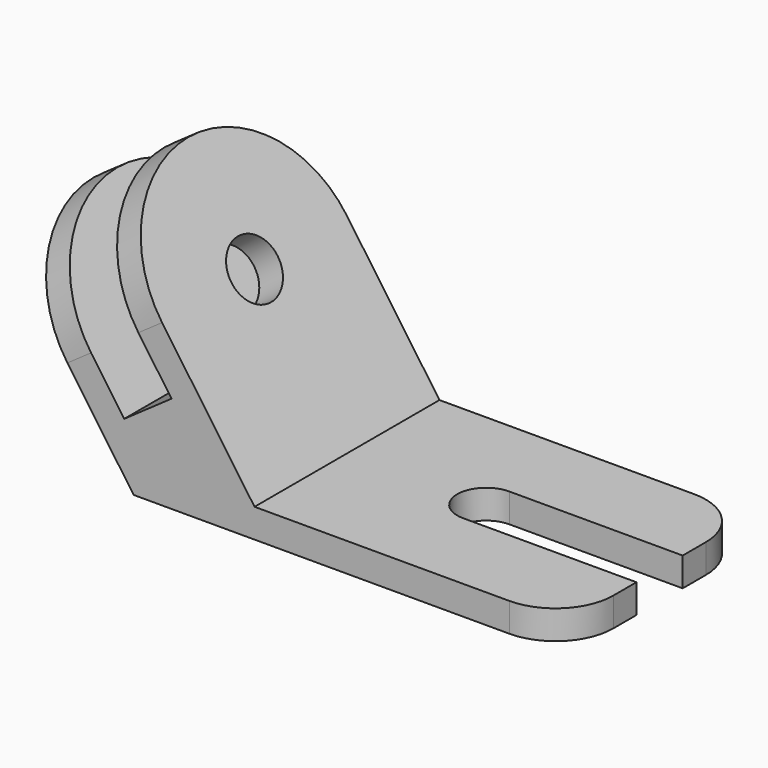
from build123d import *

# Parameters (mm, degrees)
F1_DEPTH = 80
F2_R     = 39.99999
F4_DEPTH = 25
F5_R     = 20
F6_R     = 10
F7_DEPTH = 57.1


# Not quite as in the source:
# - a fillet or chamfer is up to 0.001 mm smaller than in the source, because OpenCascade refuses the exact size


with BuildPart() as f1:
    # F0 (on Front) → F1 (new body)
    with BuildSketch(Plane.XZ):
        Polygon((-121.122470571, 65.5321635431), (-75.236355663, 0), (74.763644337, 0), (74.763644337, 10), (-25.236355663, 10), (-33.4074474946, 10), (-88.3563887995, 88.4752209972), (-96.5479092424, 82.7394566337), (-62.1333230613, 33.5903339763), (-78.5163639471, 22.1188052493), (-112.9309501282, 71.2679279066), align=None)
    extrude(amount=F1_DEPTH)

    # F2 (radius 40 in the source; OpenCascade refuses exactly that, so slightly less here)
    f2_edges = [f1.edges().sort_by_distance(p)[0] for p in [
        (-92.452149, -80, 85.607339),
        (-117.02671, -80, 68.400046),
        (-92.452149, 0, 85.607339),
        (-117.02671, 0, 68.400046),
    ]]
    fillet(f2_edges, radius=F2_R)

    # F3 (on face) → F4 (cut)
    with BuildSketch(Plane.XY.offset(10)):
        with BuildLine():
            ThreePointArc((24.763644337, -40), (21.8347121489, -47.0710678119), (14.763644337, -50))
            Line((14.763644337, -50), (134.763644337, -50))
            Line((134.763644337, -50), (134.763644337, -30))
            Line((134.763644337, -30), (14.763644337, -30))
            ThreePointArc((14.763644337, -30), (21.8347121489, -32.9289321881), (24.763644337, -40))
        make_face()
        with BuildLine():
            ThreePointArc((14.763644337, -30), (4.763644337, -40), (14.763644337, -50))
            Line((14.763644337, -50), (14.763644337, -30))
        make_face()
        with BuildLine():
            Line((14.763644337, -30), (14.763644337, -50))
            ThreePointArc((14.763644337, -50), (21.8347121489, -47.0710678119), (24.763644337, -40))
            ThreePointArc((24.763644337, -40), (21.8347121489, -32.9289321881), (14.763644337, -30))
        make_face()
    extrude(amount=-F4_DEPTH, mode=Mode.SUBTRACT)

    # F5
    f5_edges = [f1.edges().sort_by_distance(p)[0] for p in [
        (74.763644, 0, 5),
        (74.763644, -80, 5),
    ]]
    fillet(f5_edges, radius=F5_R)

    # F6 (on face) → F7 (cut)
    with BuildSketch(Plane(origin=(-17.7182706335, 0, -12.4064666616), x_dir=(0, 1, 0), z_dir=(0.8191520443, 0, 0.5735764364))):
        with Locations((-40, 83.1538007652)):
            Circle(F6_R)
    extrude(amount=-F7_DEPTH, mode=Mode.SUBTRACT)


solid = f1.part
